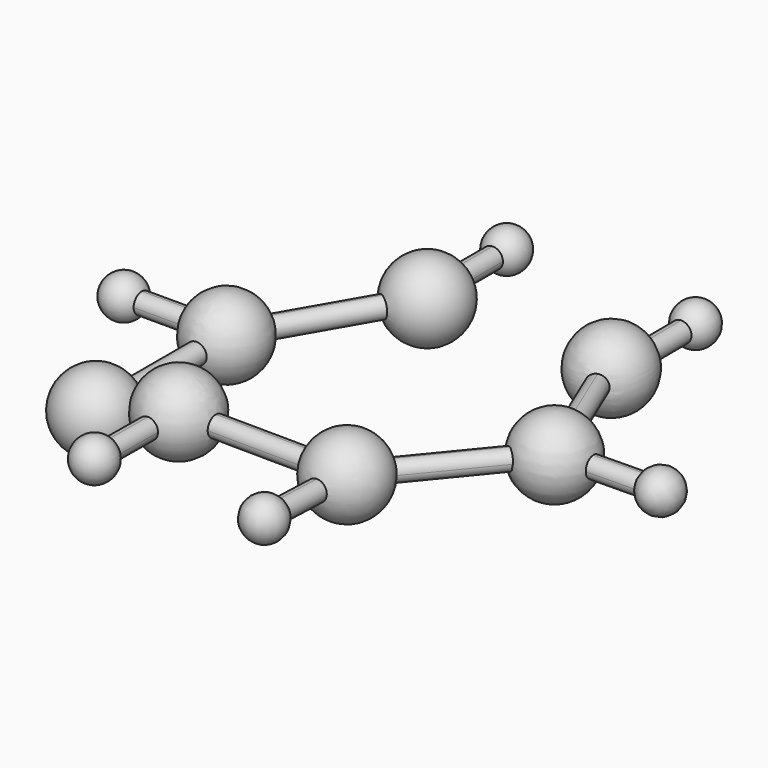
from build123d import *

# Parameters (mm, degrees)
F3_R      = 4.9859489118
F4_DEPTH  = 63.5
F9_DEPTH  = 82.55
F22_DEPTH = 82.55
F28_DEPTH = 82.55
F34_DEPTH = 82.55
F43_DEPTH = 50.8
F48_DEPTH = 50.8
F53_DEPTH = 50.8
F58_DEPTH = 50.8
F63_DEPTH = 50.8
F68_DEPTH = 50.8


# Not quite as in the source:
# - the program builds the solid bodies; features that only make, move or delete a surface that nothing else refers to are left out


with BuildPart() as f1:
    # F0 (on Front) → F1 (revolve)
    with BuildSketch(Plane.XZ):
        with BuildLine():
            Line((0, 38.1), (0, 0))
            ThreePointArc((2.03e-08, 0), (19.0500000102, 19.0500000102), (0, 38.1))
        make_face()
    revolve(axis=Axis((0, 0, 19.05), (0, 0, 1)))

    # F3 (on offset) → F4 (join)
    with BuildSketch(Plane.XZ.offset(-16.51)):
        with Locations((0, 18.6846301648)):
            Circle(F3_R)
    extrude(amount=-F4_DEPTH)

    # F5 (on face) → F6 (revolve)
    with BuildSketch(Plane(origin=(0, 80.01, 0), x_dir=(-1, 0, 0), z_dir=(0, 1, 0))):
        with BuildLine():
            Line((0, 13.698681253), (0, 0))
            ThreePointArc((0, 0), (18.9460868162, 19.05), (0, 38.1))
            Line((0, 38.1), (0, 23.6705790766))
            ThreePointArc((0, 23.6705790766), (3.5255982862, 22.210228451), (4.9859489118, 18.6846301648))
            ThreePointArc((4.9859489118, 18.6846301648), (3.5255982862, 15.1590318786), (0, 13.698681253))
        make_face()
    revolve(axis=Axis((0, 80.01, 19.05), (0, 0, -1)))

    # F8 (on line) → F9 (join)
    with BuildSketch(Plane(origin=(34.6453462784, 60.0075, 0), x_dir=(-0.8660254038, 0.5, 0), z_dir=(0.5, 0.8660254038, 0))):
        with BuildLine():
            ThreePointArc((40.2474765039, 24.0411), (35.2563765039, 19.05), (40.2474765039, 14.0589))
            Line((40.2474765039, 14.0589), (40.2474765039, 19.05))
            Line((40.2474765039, 19.05), (40.2474765039, 24.0411))
        make_face()
        with BuildLine():
            Line((40.2474765039, 19.05), (40.2474765039, 14.0589))
            ThreePointArc((40.2474765039, 14.0589), (43.7767171594, 15.5207593444), (45.2385765039, 19.05))
            ThreePointArc((45.2385765039, 19.05), (43.7767171594, 22.5792406556), (40.2474765039, 24.0411))
            Line((40.2474765039, 24.0411), (40.2474765039, 19.05))
        make_face()
    extrude(amount=F9_DEPTH)

    # F10 (on face) → F11 (revolve)
    with BuildSketch(Plane(origin=(75.9203462784, 131.4978970824, 0), x_dir=(-0.8660254038, 0.5, 0), z_dir=(0.5, 0.8660254038, 0))):
        with BuildLine():
            Line((40.2474765039, 38.1), (40.2474765039, 24.0411))
            ThreePointArc((40.2474765039, 24.0411), (43.7767171594, 22.5792406556), (45.2385765039, 19.05))
            ThreePointArc((45.2385765039, 19.05), (43.7767171594, 15.5207593444), (40.2474765039, 14.0589))
            Line((40.2474765039, 14.0589), (40.2474765039, 0))
            ThreePointArc((40.2474765039, 0), (59.2974765039, 19.05), (40.2474765039, 38.1))
        make_face()
    revolve(axis=Axis((41.0650091878, 151.6216353343, 16.55445), (0, 0, 1)))

    # F47 (on face) → F48 (join)
    with BuildSketch(Plane.XZ.offset(-151.6216353343)):
        with BuildLine():
            ThreePointArc((39.5492333709, 24.0411), (34.5581333709, 19.05), (39.5492333709, 14.0589))
            Line((39.5492333709, 14.0589), (39.5492333709, 19.05))
            Line((39.5492333709, 19.05), (39.5492333709, 24.0411))
        make_face()
        with BuildLine():
            Line((39.5492333709, 19.05), (39.5492333709, 14.0589))
            ThreePointArc((39.5492333709, 14.0589), (43.0784740265, 15.5207593444), (44.5403333709, 19.05))
            ThreePointArc((44.5403333709, 19.05), (43.0784740265, 22.5792406556), (39.5492333709, 24.0411))
            Line((39.5492333709, 24.0411), (39.5492333709, 19.05))
        make_face()
    extrude(amount=-F48_DEPTH)

    # F52 (on face) → F53 (join)
    with BuildSketch(Plane(origin=(0, 0, 0), x_dir=(0, -1, 0), z_dir=(-1, 0, 0))):
        with BuildLine():
            ThreePointArc((-75.7031248451, 19.05), (-77.1649841896, 22.5792406556), (-80.6942248451, 24.0411))
            Line((-80.6942248451, 24.0411), (-80.6942248451, 19.05))
            Line((-80.6942248451, 19.05), (-80.6942248451, 14.0589))
            ThreePointArc((-80.6942248451, 14.0589), (-77.1649841896, 15.5207593444), (-75.7031248451, 19.05))
        make_face()
        with BuildLine():
            Line((-80.6942248451, 19.05), (-80.6942248451, 24.0411))
            ThreePointArc((-80.6942248451, 24.0411), (-85.6853248451, 19.05), (-80.6942248451, 14.0589))
            Line((-80.6942248451, 14.0589), (-80.6942248451, 19.05))
        make_face()
    extrude(amount=F53_DEPTH)


with BuildPart() as f19:
    # F18 (on face) → F19 (revolve)
    with BuildSketch(Plane(origin=(116.8159328142, -12.2603782802, 11.2816771261), x_dir=(0.1034219799, 0.9945874176, 0.0099881357), z_dir=(0.9899813422, -0.1039031702, 0.0956089601))):
        with BuildLine():
            Line((162.6411825418, 25.9206794409), (162.6411825418, 11.8617794409))
            Line((162.6411825418, 11.8617794409), (162.6411825418, 6.8706794409))
            Line((162.6411825418, 6.8706794409), (162.6411825418, 1.8795794409))
            Line((162.6411825418, 1.8795794409), (162.6411825418, -12.1793205591))
            ThreePointArc((162.6411825418, -12.1793205591), (181.6911825418, 6.8706794409), (162.6411825418, 25.9206794409))
        make_face()
    revolve(axis=Axis((132.0605012608, 149.5004954579, 29.2259080463), (-0.0961292677, 0, 0.9953688582)))

    # F21 (on face) → F22 (join)
    with BuildSketch(Plane(origin=(-33.1849521527, 74.7548853547, -3.204887438), x_dir=(0.9141284845, 0.4050525361, -0.0173653906), z_dir=(0.4054246092, -0.913289555, 0.0391545008))):
        with BuildLine():
            ThreePointArc((185.9401323067, 26.9567612559), (184.4782729623, 30.4860019114), (180.9490323067, 31.9478612559))
            Line((180.9490323067, 31.9478612559), (180.9490323067, 26.9567612559))
            Line((180.9490323067, 26.9567612559), (180.9490323067, 21.9656612559))
            ThreePointArc((180.9490323067, 21.9656612559), (184.4782729623, 23.4275206003), (185.9401323067, 26.9567612559))
        make_face()
        with BuildLine():
            Line((180.9490323067, 26.9567612559), (180.9490323067, 31.9478612559))
            ThreePointArc((180.9490323067, 31.9478612559), (175.9579323067, 26.9567612559), (180.9490323067, 21.9656612559))
            Line((180.9490323067, 21.9656612559), (180.9490323067, 26.9567612559))
        make_face()
    extrude(amount=F22_DEPTH)

    # F42 (on face) → F43 (join)
    with BuildSketch(Plane(origin=(-1.3803769908, 148.2314485952, -0.1333120162), x_dir=(-0.9999566433, -0.0093118973, 8.3747e-06), z_dir=(-0.0093119011, 0.9999562389, -0.0008993111))):
        with BuildLine():
            ThreePointArc((-135.4664713144, 23.777968488), (-140.4575713144, 18.786868488), (-135.4664713144, 13.795768488))
            Line((-135.4664713144, 13.795768488), (-135.4664713144, 18.786868488))
            Line((-135.4664713144, 18.786868488), (-135.4664713144, 23.777968488))
        make_face()
        with BuildLine():
            Line((-135.4664713144, 18.786868488), (-135.4664713144, 13.795768488))
            ThreePointArc((-135.4664713144, 13.795768488), (-131.9372306589, 15.2576278324), (-130.4753713144, 18.786868488))
            ThreePointArc((-130.4753713144, 18.786868488), (-131.9372306589, 22.3161091435), (-135.4664713144, 23.777968488))
            Line((-135.4664713144, 23.777968488), (-135.4664713144, 18.786868488))
        make_face()
    extrude(amount=F43_DEPTH)

    # F44 (on face) → F45 (revolve)
    with BuildSketch(Plane(origin=(-1.8534215649, 199.0292255319, -0.1789970184), x_dir=(-0.9999566433, -0.0093118973, 8.3747e-06), z_dir=(-0.0093119011, 0.9999562389, -0.0008993111))):
        with BuildLine():
            ThreePointArc((-130.4753713144, 18.786868488), (-131.9372306589, 15.2576278324), (-135.4664713144, 13.795768488))
            Line((-135.4664713144, 13.795768488), (-135.4664713144, 8.626868488))
            ThreePointArc((-135.4664713144, 8.626868488), (-125.3064713144, 18.786868488), (-135.4664713144, 28.946868488))
            Line((-135.4664713144, 28.946868488), (-135.4664713144, 23.777968488))
            ThreePointArc((-135.4664713144, 23.777968488), (-131.9372306589, 22.3161091435), (-130.4753713144, 18.786868488))
        make_face()
    revolve(axis=Axis((133.6071763717, 200.3121400698, 23.686727332), (0, 0.0008993501, 0.9999995956)))


with BuildPart() as f24:
    # F23 (on face) → F24 (revolve)
    with BuildSketch(Plane(origin=(0.2828493408, -0.6371674109, 0.0273166071), x_dir=(0.9141284845, 0.4050525361, -0.0173653906), z_dir=(0.4054246092, -0.913289555, 0.0391545008))):
        with BuildLine():
            ThreePointArc((180.9490323067, 21.9656612559), (180.9070337049, 21.9658379618), (180.8650380769, 21.966368067))
            ThreePointArc((180.8650380769, 21.966368067), (175.9579323067, 26.9567612559), (180.8650380769, 31.9471544447))
            ThreePointArc((180.8650380769, 31.9471544447), (180.8960309257, 31.9475798324), (180.9270258185, 31.9478127407))
            Line((180.9270258185, 31.9478127407), (180.8650380769, 46.0065760836))
            ThreePointArc((180.8650380769, 46.0065760836), (161.8990785998, 26.9147640389), (180.9490323067, 7.9067612559))
            Line((180.9490323067, 7.9067612559), (180.9490323067, 21.9656612559))
        make_face()
    revolve(axis=Axis((165.6935140191, 73.4033447066, 14.3008294633), (0, -0.0428326012, -0.999082263)))


with BuildPart() as f28:
    # F27 (on face) → F28 (new body)
    with BuildSketch(Plane(origin=(92.1447490757, 126.354864431, -4.8191019369), x_dir=(0.8081778609, -0.5885106172, 0.0224454568), z_dir=(-0.5889384901, -0.8075907073, 0.0308010456))):
        with BuildLine():
            ThreePointArc((96.6197334395, 27.1637346596), (95.1578740951, 30.6929753151), (91.6286334395, 32.1548346596))
            Line((91.6286334395, 32.1548346596), (91.6286334395, 27.1637346596))
            Line((91.6286334395, 27.1637346596), (91.6286334395, 22.1726346596))
            ThreePointArc((91.6286334395, 22.1726346596), (95.1578740951, 23.634494004), (96.6197334395, 27.1637346596))
        make_face()
        with BuildLine():
            Line((91.6286334395, 27.1637346596), (91.6286334395, 32.1548346596))
            ThreePointArc((91.6286334395, 32.1548346596), (86.6375334395, 27.1637346596), (91.6286334395, 22.1726346596))
            Line((91.6286334395, 22.1726346596), (91.6286334395, 27.1637346596))
        make_face()
    extrude(amount=F28_DEPTH)

    # F29 (on face) → F30 (revolve)
    with BuildSketch(Plane(origin=(43.5278767169, 59.6882515467, -2.2764756223), x_dir=(0.8081778609, -0.5885106172, 0.0224454568), z_dir=(-0.5889384901, -0.8075907073, 0.0308010456))):
        with BuildLine():
            Line((91.7739939652, 46.2137346596), (91.7739939652, 32.1527174745))
            ThreePointArc((91.7739939652, 32.1527174745), (95.208897964, 30.6412028686), (96.6197334395, 27.1637346596))
            ThreePointArc((96.6197334395, 27.1637346596), (95.208897964, 23.6862664505), (91.7739939652, 22.1747518446))
            Line((91.7739939652, 22.1747518446), (91.7739939652, 8.1137346596))
            ThreePointArc((91.7739939652, 8.1137346596), (110.8239939652, 27.1637346596), (91.7739939652, 46.2137346596))
        make_face()
    revolve(axis=Axis((117.6975868468, 7.0765523697, 36.4455133272), (0, 0.0381117166, 0.9992734846)))

    # F33 (on face) → F34 (join)
    with BuildSketch(Plane(origin=(117.6277661319, -1.1934323085, 0.0455168226), x_dir=(-0.0101453147, -0.999948535, -3.9258e-06), z_dir=(-0.9999484601, 0.0101453155, -0.0003869365))):
        with BuildLine():
            ThreePointArc((-2.2468256599, 27.0641734824), (-3.7086850043, 30.5934141379), (-7.2379256599, 32.0552734824))
            Line((-7.2379256599, 32.0552734824), (-7.2379256599, 27.0641734824))
            Line((-7.2379256599, 27.0641734824), (-7.2379256599, 22.0730734824))
            ThreePointArc((-7.2379256599, 22.0730734824), (-3.7086850043, 23.5349328268), (-2.2468256599, 27.0641734824))
        make_face()
        with BuildLine():
            Line((-7.2379256599, 27.0641734824), (-7.2379256599, 32.0552734824))
            ThreePointArc((-7.2379256599, 32.0552734824), (-12.2290256599, 27.0641734824), (-7.2379256599, 22.0730734824))
            Line((-7.2379256599, 22.0730734824), (-7.2379256599, 27.0641734824))
        make_face()
    extrude(amount=F34_DEPTH)

    # F35 (on face) → F36 (revolve)
    with BuildSketch(Plane(origin=(35.0820207508, -0.3559365139, 0.0135752141), x_dir=(-0.0101453147, -0.999948535, -3.9258e-06), z_dir=(-0.9999484601, 0.0101453155, -0.0003869365))):
        with BuildLine():
            Line((-7.2379256599, 46.1141734824), (-7.2379256599, 32.0552734824))
            ThreePointArc((-7.2379256599, 32.0552734824), (-3.7086850043, 30.5934141379), (-2.2468256599, 27.0641734824))
            ThreePointArc((-2.2468256599, 27.0641734824), (-3.7086850043, 23.5349328268), (-7.2379256599, 22.0730734824))
            Line((-7.2379256599, 22.0730734824), (-7.2379256599, 8.0141734824))
            ThreePointArc((-7.2379256599, 8.0141734824), (11.8120743401, 27.0641734824), (-7.2379256599, 46.1141734824))
        make_face()
    revolve(axis=Axis((35.1412933691, 6.8816166459, 36.6027743718), (-0.0003869564, 0, 0.9999999251)))

    # F62 (on face) → F63 (join)
    with BuildSketch(Plane(origin=(-0.0385788318, 4.7166909916, -0.1798918846), x_dir=(-0.9999666005, -0.0081670623, 0.0003114871), z_dir=(-0.0081730001, 0.9992401094, -0.0381104437))):
        with BuildLine():
            ThreePointArc((-112.4595619573, 27.030382771), (-113.9214213017, 30.5596234266), (-117.4506619573, 32.021482771))
            Line((-117.4506619573, 32.021482771), (-117.4506619573, 27.030382771))
            Line((-117.4506619573, 27.030382771), (-117.4506619573, 22.039282771))
            ThreePointArc((-117.4506619573, 22.039282771), (-113.9214213017, 23.5011421155), (-112.4595619573, 27.030382771))
        make_face()
        with BuildLine():
            Line((-117.4506619573, 27.030382771), (-117.4506619573, 32.021482771))
            ThreePointArc((-117.4506619573, 32.021482771), (-122.4417619573, 27.030382771), (-117.4506619573, 22.039282771))
            Line((-117.4506619573, 22.039282771), (-117.4506619573, 27.030382771))
        make_face()
    extrude(amount=-F63_DEPTH)

    # F67 (on face) → F68 (join)
    with BuildSketch(Plane(origin=(0.0734310339, 7.2375531597, 2.84146e-05), x_dir=(0.999948535, -0.0101453147, -3.98e-08), z_dir=(-0.0101453147, -0.999948535, -3.9258e-06))):
        with BuildLine():
            ThreePointArc((39.8806899951, 27.2936956026), (38.4188306507, 30.8229362581), (34.8895899951, 32.2847956026))
            Line((34.8895899951, 32.2847956026), (34.8895899951, 27.2936956026))
            Line((34.8895899951, 27.2936956026), (34.8895899951, 22.3025956026))
            ThreePointArc((34.8895899951, 22.3025956026), (38.4188306507, 23.764454947), (39.8806899951, 27.2936956026))
        make_face()
        with BuildLine():
            Line((34.8895899951, 27.2936956026), (34.8895899951, 32.2847956026))
            ThreePointArc((34.8895899951, 32.2847956026), (29.8984899951, 27.2936956026), (34.8895899951, 22.3025956026))
            Line((34.8895899951, 22.3025956026), (34.8895899951, 27.2936956026))
        make_face()
    extrude(amount=F68_DEPTH)

    # F69 (on face) → F70 (revolve)
    with BuildSketch(Plane(origin=(-0.441950955, -43.5598324163, -0.0001710158), x_dir=(0.999948535, -0.0101453147, -3.98e-08), z_dir=(-0.0101453147, -0.999948535, -3.9258e-06))):
        with BuildLine():
            Line((34.8895899951, 17.1336956026), (34.8895899951, 22.3025956026))
            ThreePointArc((34.8895899951, 22.3025956026), (29.8984899951, 27.2936956026), (34.8895899951, 32.2847956026))
            Line((34.8895899951, 32.2847956026), (34.8895899951, 37.4536956026))
            ThreePointArc((34.8895899951, 37.4536956026), (24.7295899951, 27.2936956026), (34.8895899951, 17.1336956026))
        make_face()
    revolve(axis=Axis((34.4458434464, -43.9139253871, 32.3735231969), (0, -3.926e-06, 1)))


with BuildPart() as f50:
    # F49 (on face) → F50 (revolve)
    with BuildSketch(Plane(origin=(0, 202.4216353343, 0), x_dir=(-1, 0, 0), z_dir=(0, 1, 0))):
        with BuildLine():
            Line((-39.392209968, 8.89), (-39.392209968, 14.0613706431))
            ThreePointArc((-39.392209968, 14.0613706431), (-44.5403333709, 19.05), (-39.392209968, 24.0386293569))
            Line((-39.392209968, 24.0386293569), (-39.392209968, 29.21))
            ThreePointArc((-39.392209968, 29.21), (-49.552209968, 19.05), (-39.392209968, 8.89))
        make_face()
    revolve(axis=Axis((39.392209968, 202.4216353343, 13.97), (0, 0, -1)))


with BuildPart() as f55:
    # F54 (on face) → F55 (revolve)
    with BuildSketch(Plane(origin=(-50.8, 0, 0), x_dir=(0, -1, 0), z_dir=(-1, 0, 0))):
        with BuildLine():
            Line((-80.6942248451, 29.21), (-80.6942248451, 24.0411))
            ThreePointArc((-80.6942248451, 24.0411), (-77.1649841896, 22.5792406556), (-75.7031248451, 19.05))
            ThreePointArc((-75.7031248451, 19.05), (-77.1649841896, 15.5207593444), (-80.6942248451, 14.0589))
            Line((-80.6942248451, 14.0589), (-80.6942248451, 8.89))
            ThreePointArc((-80.6942248451, 8.89), (-70.5342248451, 19.05), (-80.6942248451, 29.21))
        make_face()
    revolve(axis=Axis((-50.8, 80.6942248451, 24.13), (0, 0, 1)))


with BuildPart() as f58:
    # F57 (on face) → F58 (new body)
    with BuildSketch(Plane(origin=(166.8156591609, 2.6697544925, -0.1144575715), x_dir=(0.0160021631, -0.9998719571, -1.09796e-05), z_dir=(-0.9998717218, -0.0160021669, 0.000686044))):
        with BuildLine():
            ThreePointArc((-71.8198940158, 29.3617421461), (-76.8109940158, 24.3706421461), (-71.8198940158, 19.3795421461))
            Line((-71.8198940158, 19.3795421461), (-71.8198940158, 24.3706421461))
            Line((-71.8198940158, 24.3706421461), (-71.8198940158, 29.3617421461))
        make_face()
        with BuildLine():
            Line((-71.8198940158, 24.3706421461), (-71.8198940158, 19.3795421461))
            ThreePointArc((-71.8198940158, 19.3795421461), (-68.2906533602, 20.8414014905), (-66.8287940158, 24.3706421461))
            ThreePointArc((-66.8287940158, 24.3706421461), (-68.2906533602, 27.8998828017), (-71.8198940158, 29.3617421461))
            Line((-71.8198940158, 29.3617421461), (-71.8198940158, 24.3706421461))
        make_face()
    extrude(amount=-F58_DEPTH)


with BuildPart() as f60:
    # F59 (on face) → F60 (revolve)
    with BuildSketch(Plane(origin=(217.6091426269, 3.4826645716, -0.1493086088), x_dir=(-0.0160021631, 0.9998719571, 1.09796e-05), z_dir=(0.9998717218, 0.0160021669, -0.000686044))):
        with BuildLine():
            Line((61.6598940158, 24.3706421461), (66.8287940158, 24.3706421461))
            ThreePointArc((66.8287940158, 24.3706421461), (71.8198940158, 29.3617421461), (76.8109940158, 24.3706421461))
            Line((76.8109940158, 24.3706421461), (81.9798940158, 24.3706421461))
            ThreePointArc((81.9798940158, 24.3706421461), (71.8198940158, 34.5306421461), (61.6598940158, 24.3706421461))
        make_face()
    revolve(axis=Axis((216.5578814296, 70.2140130198, 24.2220605778), (0.0160021631, -0.9998719571, -1.09796e-05)))


with BuildPart() as f65:
    # F64 (on face) → F65 (revolve)
    with BuildSketch(Plane(origin=(0.3766095752, -46.0447065638, 1.7561186551), x_dir=(0.9999666005, 0.0081670623, -0.0003114871), z_dir=(0.0081730001, -0.9992401094, 0.0381104437))):
        with BuildLine():
            Line((117.4506619573, 37.190382771), (117.4506619573, 32.021482771))
            ThreePointArc((117.4506619573, 32.021482771), (120.9799026128, 30.5596234266), (122.4417619573, 27.030382771))
            ThreePointArc((122.4417619573, 27.030382771), (120.9799026128, 23.5011421155), (117.4506619573, 22.039282771))
            Line((117.4506619573, 22.039282771), (117.4506619573, 16.870382771))
            ThreePointArc((117.4506619573, 16.870382771), (127.6106619573, 27.030382771), (117.4506619573, 37.190382771))
        make_face()
    revolve(axis=Axis((117.8233487364, -44.2489129194, 23.6539697734), (0, -0.0381117166, -0.9992734846)))


solid = Compound([f1.part, f19.part, f24.part, f28.part, f50.part, f55.part, f58.part, f60.part, f65.part])
